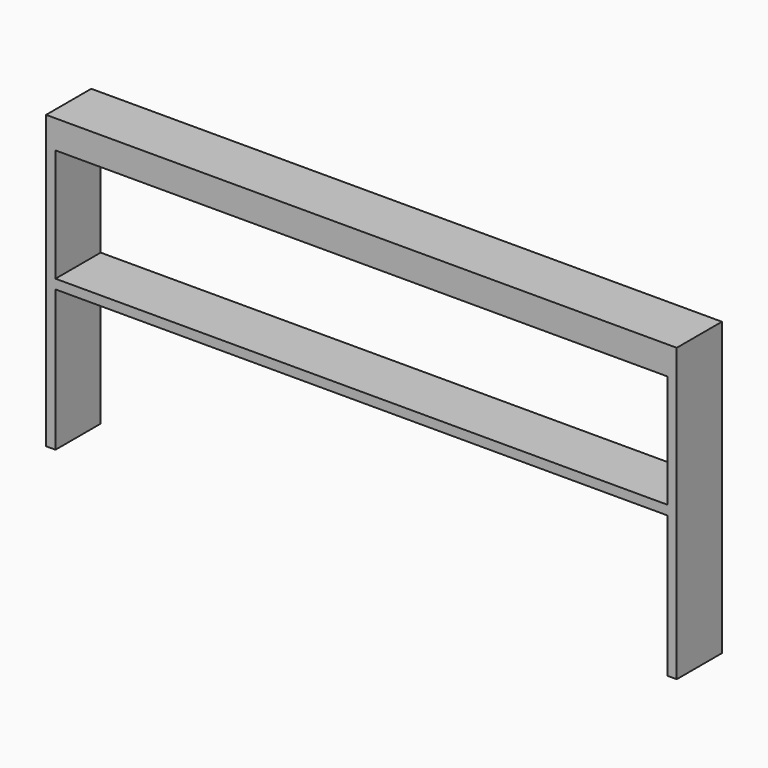
from build123d import *

# Parameters (mm, degrees)
F0_W      = 1651
F0_H      = 25.4
F1_DEPTH  = 152.4
F0_H_2    = 50.8
F2_DEPTH  = 25.4
F3_START  = 101.6
F2_FACE_W = 1651
F2_FACE_H = 50.8
F3_DEPTH  = 25.4


# Not quite as in the source:
# - a feature names something its author has since deleted; it is built from what else it names


with BuildPart() as f1:
    # F0 (on Front) → F1 (new body)
    with BuildSketch(Plane.XZ):
        Polygon((-850.9, 368.3), (-850.9, -393.7), (-825.5, -393.7), (-825.5, -12.7), (-825.5, 12.7), (-825.5, 317.5), (-825.5, 368.3), align=None)
        Polygon((-850.9, 393.7), (-850.9, 368.3), (-825.5, 368.3), (825.5, 368.3), (850.9, 368.3), (850.9, 393.7), align=None)
        Polygon((825.5, 12.7), (825.5, -12.7), (825.5, -393.7), (850.9, -393.7), (850.9, 368.3), (825.5, 368.3), (825.5, 317.5), align=None)
        Rectangle(F0_W, F0_H)
    extrude(amount=F1_DEPTH)

    # F0 (on Front) → F2 (join)
    with BuildSketch(Plane.XZ):
        with Locations((0, 342.9)):
            Rectangle(F0_W, F0_H_2)
    extrude(amount=F2_DEPTH)

    # F2_face (on face) → F3 (join)
    with BuildSketch(Plane(origin=(0, -25.4, 342.9), x_dir=(1, 0, 0), z_dir=(0, -1, 0)).offset(F3_START)):
        Rectangle(F2_FACE_W, F2_FACE_H)
    extrude(amount=F3_DEPTH)


solid = f1.part
